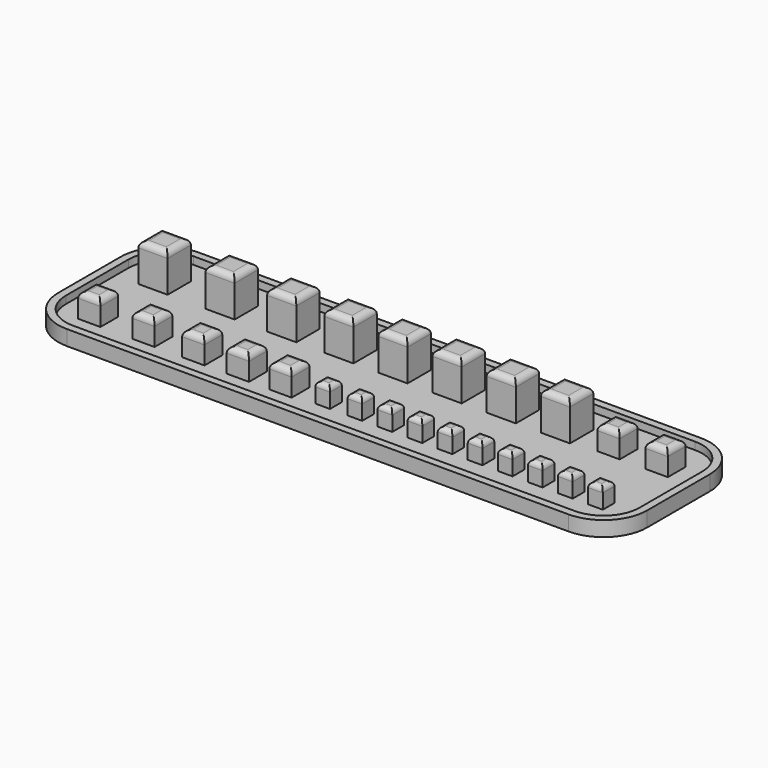
from build123d import *

# Parameters (mm, degrees)
F0_W      = 242.3795
F0_H      = 63.5
F1_DEPTH  = 3.175
F2_W      = 12.319
F2_H      = 12.319
F3_DEPTH  = 16.002
F4_W      = 9.398
F4_H      = 9.398
F5_DEPTH  = 10.16
F6_R      = 15.24
F7_R      = 2.54
F8_R      = 2.54
F9_W      = 6.223
F9_H      = 6.223
F10_DEPTH = 8.255
F11_R     = 2.032
F13_DEPTH = 6.35


# Not quite as in the source:
# - a feature names something its author has since deleted; it is built from what else it names


with BuildPart() as f1:
    # F0 (on Top) → F1 (new body)
    with BuildSketch(Plane.XY):
        with Locations((111.47425, -22.0218)):
            Rectangle(F0_W, F0_H)
    extrude(amount=-F1_DEPTH)

    # F2 (on Top) → F3 (join)
    with BuildSketch(Plane.XY):
        with Locations((6.1595, -6.1595)):
            Rectangle(F2_W, F2_H)
        with Locations((34.4805, -6.1595)):
            Rectangle(F2_W, F2_H)
        with Locations((60.5155, -6.1595)):
            Rectangle(F2_W, F2_H)
        with Locations((84.6455, -6.1595)):
            Rectangle(F2_W, F2_H)
        with Locations((107.5055, -6.1595)):
            Rectangle(F2_W, F2_H)
        with Locations((130.3655, -6.1595)):
            Rectangle(F2_W, F2_H)
        with Locations((153.2255, -6.1595)):
            Rectangle(F2_W, F2_H)
        with Locations((176.0855, -6.1595)):
            Rectangle(F2_W, F2_H)
    extrude(amount=F3_DEPTH)

    # F4 (on face) → F5 (join)
    with BuildSketch(Plane.XY):
        with Locations((48.641, -39.4335)):
            Rectangle(F4_W, F4_H)
        with Locations((67.437, -39.4335)):
            Rectangle(F4_W, F4_H)
        with Locations((85.471, -39.4335)):
            Rectangle(F4_W, F4_H)
        with Locations((27.559, -39.4335)):
            Rectangle(F4_W, F4_H)
        with Locations((4.699, -39.4335)):
            Rectangle(F4_W, F4_H)
        with Locations((197.485, -6.2865)):
            Rectangle(F4_W, F4_H)
        with Locations((217.805, -6.2865)):
            Rectangle(F4_W, F4_H)
    extrude(amount=F5_DEPTH)

    # F6
    f6_edges = [f1.edges().sort_by_distance(p)[0] for p in [
        (-9.7155, 9.7282, -1.5875),
        (232.664, 9.7282, -1.5875),
        (232.664, -53.7718, -1.5875),
        (-9.7155, -53.7718, -1.5875),
    ]]
    fillet(f6_edges, radius=F6_R)

    # F7
    f7_edges = [f1.edges().sort_by_distance(p)[0] for p in [
        (6.1595, 0, 16.002),
        (0, -6.1595, 16.002),
        (6.1595, -12.319, 16.002),
        (12.319, -6.1595, 16.002),
        (34.4805, 0, 16.002),
        (28.321, -6.1595, 16.002),
        (34.4805, -12.319, 16.002),
        (40.64, -6.1595, 16.002),
        (60.5155, 0, 16.002),
        (54.356, -6.1595, 16.002),
        (60.5155, -12.319, 16.002),
        (66.675, -6.1595, 16.002),
        (84.6455, 0, 16.002),
        (78.486, -6.1595, 16.002),
        (84.6455, -12.319, 16.002),
        (90.805, -6.1595, 16.002),
        (107.5055, 0, 16.002),
        (101.346, -6.1595, 16.002),
        (107.5055, -12.319, 16.002),
        (113.665, -6.1595, 16.002),
        (130.3655, 0, 16.002),
        (124.206, -6.1595, 16.002),
        (130.3655, -12.319, 16.002),
        (136.525, -6.1595, 16.002),
        (153.2255, 0, 16.002),
        (147.066, -6.1595, 16.002),
        (153.2255, -12.319, 16.002),
        (159.385, -6.1595, 16.002),
        (176.0855, 0, 16.002),
        (169.926, -6.1595, 16.002),
        (176.0855, -12.319, 16.002),
        (182.245, -6.1595, 16.002),
    ]]
    fillet(f7_edges, radius=F7_R)

    # F8
    f8_edges = [f1.edges().sort_by_distance(p)[0] for p in [
        (4.699, -34.7345, 10.16),
        (0, -39.4335, 10.16),
        (4.699, -44.1325, 10.16),
        (9.398, -39.4335, 10.16),
        (27.559, -34.7345, 10.16),
        (22.86, -39.4335, 10.16),
        (27.559, -44.1325, 10.16),
        (32.258, -39.4335, 10.16),
        (48.641, -34.7345, 10.16),
        (43.942, -39.4335, 10.16),
        (48.641, -44.1325, 10.16),
        (53.34, -39.4335, 10.16),
        (67.437, -34.7345, 10.16),
        (62.738, -39.4335, 10.16),
        (67.437, -44.1325, 10.16),
        (72.136, -39.4335, 10.16),
        (85.471, -34.7345, 10.16),
        (80.772, -39.4335, 10.16),
        (85.471, -44.1325, 10.16),
        (90.17, -39.4335, 10.16),
        (197.485, -1.5875, 10.16),
        (192.786, -6.2865, 10.16),
        (197.485, -10.9855, 10.16),
        (202.184, -6.2865, 10.16),
        (217.805, -1.5875, 10.16),
        (213.106, -6.2865, 10.16),
        (217.805, -10.9855, 10.16),
        (222.504, -6.2865, 10.16),
    ]]
    fillet(f8_edges, radius=F8_R)

    # F9 (on face) → F10 (join)
    with BuildSketch(Plane.XY):
        with Locations((101.981, -39.4335)):
            Rectangle(F9_W, F9_H)
        with Locations((115.57, -39.4335)):
            Rectangle(F9_W, F9_H)
        with Locations((128.27, -39.4335)):
            Rectangle(F9_W, F9_H)
        with Locations((140.97, -39.4335)):
            Rectangle(F9_W, F9_H)
        with Locations((153.67, -39.4335)):
            Rectangle(F9_W, F9_H)
        with Locations((166.37, -39.4335)):
            Rectangle(F9_W, F9_H)
        with Locations((179.07, -39.4335)):
            Rectangle(F9_W, F9_H)
        with Locations((191.77, -39.4335)):
            Rectangle(F9_W, F9_H)
        with Locations((204.47, -39.4335)):
            Rectangle(F9_W, F9_H)
        with Locations((217.17, -39.4335)):
            Rectangle(F9_W, F9_H)
    extrude(amount=F10_DEPTH)

    # F11
    f11_edges = [f1.edges().sort_by_distance(p)[0] for p in [
        (101.981, -36.322, 8.255),
        (98.8695, -39.4335, 8.255),
        (101.981, -42.545, 8.255),
        (105.0925, -39.4335, 8.255),
        (115.57, -36.322, 8.255),
        (112.4585, -39.4335, 8.255),
        (115.57, -42.545, 8.255),
        (118.6815, -39.4335, 8.255),
        (128.27, -36.322, 8.255),
        (125.1585, -39.4335, 8.255),
        (128.27, -42.545, 8.255),
        (131.3815, -39.4335, 8.255),
        (140.97, -36.322, 8.255),
        (137.8585, -39.4335, 8.255),
        (140.97, -42.545, 8.255),
        (144.0815, -39.4335, 8.255),
        (153.67, -36.322, 8.255),
        (150.5585, -39.4335, 8.255),
        (153.67, -42.545, 8.255),
        (156.7815, -39.4335, 8.255),
        (166.37, -36.322, 8.255),
        (163.2585, -39.4335, 8.255),
        (166.37, -42.545, 8.255),
        (169.4815, -39.4335, 8.255),
        (179.07, -36.322, 8.255),
        (175.9585, -39.4335, 8.255),
        (179.07, -42.545, 8.255),
        (182.1815, -39.4335, 8.255),
        (191.77, -36.322, 8.255),
        (188.6585, -39.4335, 8.255),
        (191.77, -42.545, 8.255),
        (194.8815, -39.4335, 8.255),
        (204.47, -36.322, 8.255),
        (201.3585, -39.4335, 8.255),
        (204.47, -42.545, 8.255),
        (207.5815, -39.4335, 8.255),
        (217.17, -36.322, 8.255),
        (214.0585, -39.4335, 8.255),
        (217.17, -42.545, 8.255),
        (220.2815, -39.4335, 8.255),
    ]]
    fillet(f11_edges, radius=F11_R)

    # F12 (on face) → F13 (join)
    with BuildSketch(Plane(origin=(0, 0, -3.175), x_dir=(1, 0, 0), z_dir=(0, 0, -1))):
        with BuildLine():
            Line((217.424, 56.9468), (5.5245, 56.9468))
            ThreePointArc((5.5245, 56.9468), (-7.4968713756, 51.5531713756), (-12.8905, 38.5318))
            Line((-12.8905, 38.5318), (-12.8905, 5.5118))
            ThreePointArc((-12.8905, 5.5118), (-7.4968713756, -7.5095713756), (5.5245, -12.9032))
            Line((5.5245, -12.9032), (217.424, -12.9032))
            ThreePointArc((217.424, -12.9032), (230.4453713756, -7.5095713756), (235.839, 5.5118))
            Line((235.839, 5.5118), (235.839, 38.5318))
            ThreePointArc((235.839, 38.5318), (230.4453713756, 51.5531713756), (217.424, 56.9468))
        make_face()
        with BuildLine():
            Line((217.424, -9.7282), (5.5245, -9.7282))
            ThreePointArc((5.5245, -9.7282), (-5.2518073453, -5.2645073453), (-9.7155, 5.5118))
            Line((-9.7155, 5.5118), (-9.7155, 38.5318))
            ThreePointArc((-9.7155, 38.5318), (-5.2518073453, 49.3081073453), (5.5245, 53.7718))
            Line((5.5245, 53.7718), (217.424, 53.7718))
            ThreePointArc((217.424, 53.7718), (228.2003073453, 49.3081073453), (232.664, 38.5318))
            Line((232.664, 38.5318), (232.664, 5.5118))
            ThreePointArc((232.664, 5.5118), (228.2003073453, -5.2645073453), (217.424, -9.7282))
        make_face(mode=Mode.SUBTRACT)
    extrude(amount=-F13_DEPTH)


solid = f1.part
